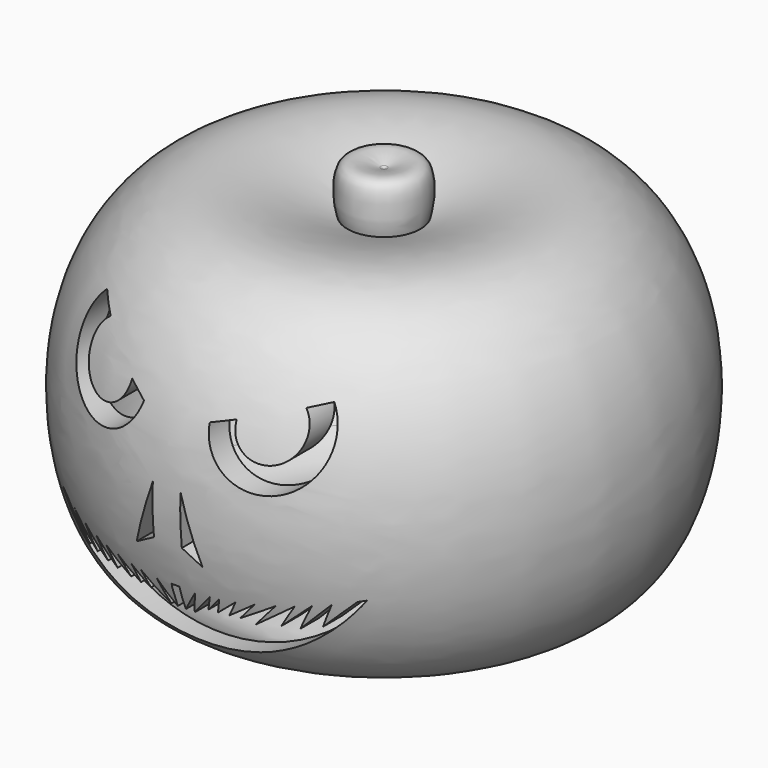
from build123d import *

# Parameters (mm, degrees)
F3_DEPTH = 25.4


# Not quite as in the source:
# - a feature names something its author has since deleted; it is built from what else it names


with BuildPart() as f1:
    # F0 (on Front) → F1 (revolve)
    with BuildSketch(Plane.XZ):
        with BuildLine():
            add(Edge.make_bspline(
                [(-9.720892116, 11.7351212028), (-9.6590186821, 11.7283836809), (-9.4396738554, 11.7360560454), (-9.5153778587, 11.9904832515), (-9.5736505464, 12.1863270178)],
                knots=[0.8567009755, 0.8567009755, 0.8567009755, 0.8567009755, 0.8896964632, 1, 1, 1, 1], degree=3))
            add(Edge.make_bspline(
                [(-9.5736505464, 12.1863270178), (-10.6666631758, 12.5697912998), (-12.8535529972, 13.3370231804), (-12.4778606487, 9.4990431586), (-12.231747593, 8.798820588)],
                knots=[0, 0, 0, 0, 0.403533425, 0.807386041, 0.807386041, 0.807386041, 0.807386041], degree=3))
            add(Edge.make_bspline(
                [(-12.2317475816, 8.7988205971), (-15.8222950063, 10.1452037231), (-23.2569270221, 12.8022862545), (-32.2778207644, 1.9872480307), (-28.6086021959, -19.5198789177), (-15.9116846694, -15.9731174733), (-9.5736505464, -14.2026487738)],
                knots=[0.0069469557, 0.0069469557, 0.0069469557, 0.0069469557, 0.2213400288, 0.4525400575, 0.7267195137, 1, 1, 1, 1], degree=3))
            Line((-9.5736505464, -14.2026487738), (-9.5736505464, -12.9766762257))
            add(Edge.make_bspline(
                [(-25.3317989409, -14.129858464), (-24.8068212673, -14.4068742314), (-23.7060427055, -14.9877237292), (-21.5749292194, -15.7962292432), (-18.6495786438, -15.206467766), (-15.0881032424, -14.9086527805), (-11.55985804, -13.6725397179), (-9.5736505464, -12.9766762257)],
                knots=[0, 0, 0, 0, 0.1525656923, 0.319901306, 0.5112059253, 0.7248358891, 1, 1, 1, 1], degree=3))
            ThreePointArc((-25.3317989409, -14.129858464), (-28.6194152979, -1.8253104494), (-22.6186513901, 9.4086183235))
            add(Edge.make_bspline(
                [(-22.6186513901, 9.4086183235), (-22.3655846497, 9.6772071829), (-21.3146492859, 10.7926027905), (-14.6405881811, 8.5406198758), (-9.5736505464, 6.8309176713)],
                knots=[0, 0, 0, 0, 0.2408014318, 1, 1, 1, 1], degree=3))
            add(Edge.make_bspline(
                [(-9.5736505464, 6.8309176713), (-10.2234278845, 7.3254825573), (-11.4869483986, 8.287185655), (-11.5170338603, 10.3186632878), (-11.3441864921, 12.3123398514), (-10.0258638395, 11.7683301834), (-9.720892116, 11.7351212028)],
                knots=[0, 0, 0, 0, 0.250841613, 0.4877725109, 0.6940675134, 0.8567009755, 0.8567009755, 0.8567009755, 0.8567009755], degree=3))
        make_face()
        with BuildLine():
            add(Edge.make_bspline(
                [(-12.231747593, 8.798820588), (-12.1894295385, 8.6784204051), (-12.0672758209, 8.4444662202), (-11.9546861362, 8.5806869743), (-11.8826869875, 8.6677977815)],
                knots=[0.807386041, 0.807386041, 0.807386041, 0.807386041, 0.8768267172, 1, 1, 1, 1], degree=3))
            add(Edge.make_bspline(
                [(-11.8826869875, 8.6677977815), (-11.9990452233, 8.7114958354), (-12.115403459, 8.7551938893), (-12.2317475816, 8.7988205971)],
                knots=[0, 0, 0, 0, 0.0069469557, 0.0069469557, 0.0069469557, 0.0069469557], degree=3))
        make_face(mode=Mode.SUBTRACT)
        with BuildLine():
            Line((-9.3187112361, 12.0893660933), (-9.5736505464, 12.1863270178))
            add(Edge.make_bspline(
                [(-9.720892116, 11.7351212028), (-9.6590186821, 11.7283836809), (-9.4396738554, 11.7360560454), (-9.5153778587, 11.9904832515), (-9.5736505464, 12.1863270178)],
                knots=[0.8567009755, 0.8567009755, 0.8567009755, 0.8567009755, 0.8896964632, 1, 1, 1, 1], degree=3))
            Line((-9.720892116, 11.7351212028), (-9.3187112361, 11.5901101381))
            Line((-9.3187112361, 11.5901101381), (-9.3187112361, 12.0893660933))
        make_face()
        with BuildLine():
            add(Edge.make_bspline(
                [(-11.8826869875, 8.6677977815), (-11.9990452233, 8.7114958354), (-12.115403459, 8.7551938893), (-12.2317475816, 8.7988205971)],
                knots=[0, 0, 0, 0, 0.0069469557, 0.0069469557, 0.0069469557, 0.0069469557], degree=3))
            add(Edge.make_bspline(
                [(-12.231747593, 8.798820588), (-12.1894295385, 8.6784204051), (-12.0672758209, 8.4444662202), (-11.9546861362, 8.5806869743), (-11.8826869875, 8.6677977815)],
                knots=[0.807386041, 0.807386041, 0.807386041, 0.807386041, 0.8768267172, 1, 1, 1, 1], degree=3))
        make_face()
    revolve(axis=Axis((-9.3187112361, 0, 11.8397381157), (0, 0, -1)))

    # F2 (on Front) → F3 (cut)
    with BuildSketch(Plane.XZ):
        with BuildLine():
            Line((-17.6470892382, 5.8834053887), (-19.0875875563, 6.7421640375))
            ThreePointArc((-19.0875875563, 6.7421640375), (-18.4162875763, 0.4277474899), (-12.542411685, 2.8402321041))
            Line((-12.542411685, 2.8402321041), (-13.9543497699, 3.6819644593))
            ThreePointArc((-13.9543497699, 3.6819644593), (-17.5795365416, 1.7988629219), (-17.6470892382, 5.8834053887))
        make_face()
        with BuildLine():
            Line((-5.4598796671, 3.6619777803), (-7.2300815478, 3.0728209522))
            ThreePointArc((-7.2300815478, 3.0728209522), (-2.0108350774, -0.5440791406), (0, 5.479129497))
            Line((0, 5.479129497), (-1.4349934442, 5.0015364071))
            ThreePointArc((-1.4349934442, 5.0015364071), (-2.4581103196, 1.3591917594), (-5.4598796671, 3.6619777803))
        make_face()
        Polygon((-11.0030537471, -5.8786282316), (-11.0030537471, -1.9199585076), (-12.6586532444, -6.8428988422), align=None)
        Polygon((-7.2646159679, -6.8428988422), (-8.7376036992, -1.9199585076), (-8.7376036992, -5.8786282316), align=None)
        with BuildLine():
            ThreePointArc((-21.23939498, -7.7997265919), (-21.5642286708, -7.7199956019), (-21.8885075301, -7.6380372047))
            ThreePointArc((-21.8885075301, -7.6380372047), (-9.545048066, -13.9897187449), (2.7412043419, -7.5280740857))
            ThreePointArc((2.7412043419, -7.5280740857), (2.4868724044, -7.5949750605), (2.2321831736, -7.6605026925))
            Line((2.2321831736, -7.6605026925), (0, -9.862896055))
            Line((0, -9.862896055), (0.8131507344, -7.9989894423))
            Line((0.8131507344, -7.9989894423), (-1.4080617111, -10.2617209777))
            Line((-1.4080617111, -10.2617209777), (-0.337813808, -8.2408511617))
            Line((-0.337813808, -8.2408511617), (-2.5645566639, -10.2617209777))
            Line((-2.5645566639, -10.2617209777), (-1.3722431055, -8.4336452967))
            Line((-1.3722431055, -8.4336452967), (-4.2601174528, -10.5272321251))
            Line((-4.2601174528, -10.5272321251), (-2.5697043411, -8.6281462356))
            Line((-2.5697043411, -8.6281462356), (-5.2292268711, -10.2617209777))
            Line((-5.2292268711, -10.2617209777), (-3.9400693354, -8.8134235951))
            Line((-3.9400693354, -8.8134235951), (-5.9941634536, -10.2617209777))
            Line((-5.9941634536, -10.2617209777), (-5.2335678583, -8.952167619))
            Line((-5.2335678583, -8.952167619), (-6.7917467095, -10.2617209777))
            Line((-6.7917467095, -10.2617209777), (-6.4188276828, -9.0487503644))
            Line((-6.4188276828, -9.0487503644), (-7.4985163058, -10.2617209777))
            Line((-7.4985163058, -10.2617209777), (-7.1049828011, -9.0913834251))
            Line((-7.1049828011, -9.0913834251), (-8.7376036992, -10.9255429502))
            Line((-8.7376036992, -10.9255429502), (-8.2183042541, -9.1439904645))
            Line((-8.2183042541, -9.1439904645), (-9.4388024881, -10.9255429502))
            Line((-9.4388024881, -10.9255429502), (-9.4388024881, -9.0814009309))
            Line((-9.4388024881, -9.0814009309), (-10.0646987557, -9.0814009309))
            Line((-10.0646987557, -9.0814009309), (-10.0959930569, -9.3317590654))
            Line((-10.0959930569, -9.3317590654), (-10.0959930569, -10.9255429502))
            Line((-10.0959930569, -10.9255429502), (-11.3790798932, -9.0814009309))
            Line((-11.3790798932, -9.0814009309), (-10.6216668073, -10.9255429502))
            Line((-10.6216668073, -10.9255429502), (-12.7505537679, -9.0747226052))
            Line((-12.7505537679, -9.0747226052), (-12.1754324064, -10.2617209777))
            Line((-12.1754324064, -10.2617209777), (-13.6098035416, -9.0147016062))
            Line((-13.6098035416, -9.0147016062), (-13.0926528946, -10.2617209777))
            Line((-13.0926528946, -10.2617209777), (-14.9344921101, -8.8921847252))
            Line((-14.9344921101, -8.8921847252), (-14.0497516841, -10.2617209777))
            Line((-14.0497516841, -10.2617209777), (-16.2030621966, -8.7405325467))
            Line((-16.2030621966, -8.7405325467), (-15.4455220327, -10.2617209777))
            Line((-15.4455220327, -10.2617209777), (-17.260157616, -8.5882797056))
            Line((-17.260157616, -8.5882797056), (-16.5222585201, -10.2617209777))
            Line((-16.5222585201, -10.2617209777), (-18.6142992725, -8.3584879409))
            Line((-18.6142992725, -8.3584879409), (-17.7585128695, -10.2218389511))
            Line((-17.7585128695, -10.2218389511), (-20.0031616776, -8.0816983925))
            Line((-20.0031616776, -8.0816983925), (-18.7953710556, -10.2218389511))
            Line((-18.7953710556, -10.2218389511), (-21.23939498, -7.7997265919))
        make_face()
    extrude(amount=F3_DEPTH, mode=Mode.SUBTRACT)


solid = f1.part
